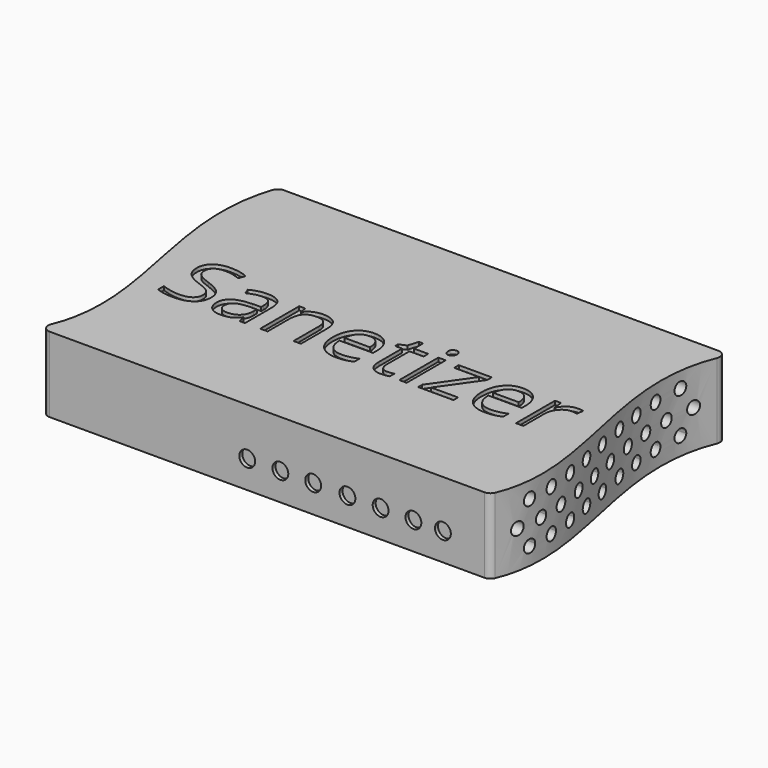
from build123d import *

# Parameters (mm, degrees)
F1_DEPTH      = 25.4
F2_R          = 2.54
F3_TEXT_SIZE  = 30.7263651242
F4_DEPTH      = 1.27
F5_R          = 2.1391280129
F6_DEPTH      = 87.376
F6_DEPTH_BACK = 113.538
F7_W          = 14.690361917
F7_H          = 8.7442630902
F7_W_2        = 13.8159319758
F7_W_3        = 14.3405906856
F7_W_4        = 15.2150169015
F7_W_5        = 12.766623171
F7_H_2        = 4.8967869952
F7_W_6        = 21.1611157283
F7_R          = 3.9572028388
F8_DEPTH      = 7.62
F9_R          = 2.6752298393
F10_DEPTH     = 1.27


# Not quite as in the source:
# - Text() gives the source's letters only with a copy of the font that has no kerning and outlines rounded to 1/6400 em; it was checked with that copy


with BuildPart() as f1:
    # F0 (on Top) → F1 (new body)
    with BuildSketch(Plane.XY):
        with BuildLine():
            add(Edge.make_bspline(
                [(-45.4201986909, 65.6159471944), (-58.06190148, 32.6160974801), (-29.9053769559, -7.6075084507), (-45.4201986909, -35.9840528056)],
                knots=[0, 0, 0, 0, 101.6, 101.6, 101.6, 101.6], degree=3))
            Line((-45.4201986909, -35.9840528056), (106.9798013091, -35.9840528056))
            add(Edge.make_bspline(
                [(106.9798013091, 65.6159471944), (90.3426812113, 34.0577052146), (120.670825243, -8.1321643665), (106.9798013091, -35.9840528056)],
                knots=[0, 0, 0, 0, 101.6, 101.6, 101.6, 101.6], degree=3))
            Line((106.9798013091, 65.6159471944), (-45.4201986909, 65.6159471944))
        make_face()
    extrude(amount=F1_DEPTH)

    # F2
    f2_edges = [f1.edges().sort_by_distance(p)[0] for p in [
        (106.979801, 65.615947, 12.7),
        (-45.420199, -35.984053, 12.7),
        (-45.420199, 65.615947, 12.7),
        (106.979801, -35.984053, 12.7),
    ]]
    fillet(f2_edges, radius=F2_R)

    # F3 (on face) → F4 (cut)
    with BuildSketch(Plane.XY.offset(25.4)):
        with Locations((-35.7243866998, 0)):
            Text('Sanetizer', F3_TEXT_SIZE, font='Open Sans', text_align=(TextAlign.LEFT, TextAlign.BOTTOM))
    extrude(amount=-F4_DEPTH, mode=Mode.SUBTRACT)

    # F5 (on Right) → F6 (cut, two sides)
    with BuildSketch(Plane.YZ) as f6_sk:
        with BuildLine():
            ThreePointArc((-25.4598658399, 12.6498732716), (-27.5989938527, 14.7890012844), (-29.7381218656, 12.6498732716))
            Line((-29.7381218656, 12.6498732716), (-25.4598658399, 12.6498732716))
        make_face()
        with BuildLine():
            ThreePointArc((57.1315141528, 12.8702148795), (54.882068538, 15.0064963877), (52.8646365703, 12.6498732716))
            Line((52.8646365703, 12.6498732716), (57.1201357096, 12.6498732716))
            ThreePointArc((57.1201357096, 12.6498732716), (57.1286676481, 12.7598972776), (57.1315141528, 12.8702148795))
        make_face()
        with BuildLine():
            Line((57.1201357096, 12.6498732716), (52.8646365703, 12.6498732716))
            ThreePointArc((52.8646365703, 12.6498732716), (54.9923861399, 10.7310868667), (57.1201357096, 12.6498732716))
        make_face()
        with BuildLine():
            ThreePointArc((47.2161371394, 12.6498732716), (45.0770091265, 14.7890012844), (42.9378811137, 12.6498732716))
            Line((42.9378811137, 12.6498732716), (47.2161371394, 12.6498732716))
        make_face()
        with BuildLine():
            Line((47.2161371394, 12.6498732716), (42.9378811137, 12.6498732716))
            ThreePointArc((42.9378811137, 12.6498732716), (45.0770091265, 10.5107452587), (47.2161371394, 12.6498732716))
        make_face()
        with BuildLine():
            ThreePointArc((38.182130283, 12.6498732716), (36.0430022702, 14.7890012844), (33.9038742573, 12.6498732716))
            Line((33.9038742573, 12.6498732716), (38.182130283, 12.6498732716))
        make_face()
        with BuildLine():
            Line((38.182130283, 12.6498732716), (33.9038742573, 12.6498732716))
            ThreePointArc((33.9038742573, 12.6498732716), (36.0430022702, 10.5107452587), (38.182130283, 12.6498732716))
        make_face()
        with BuildLine():
            ThreePointArc((29.2582979559, 12.6498732716), (27.119169943, 14.7890012844), (24.9800419302, 12.6498732716))
            Line((24.9800419302, 12.6498732716), (29.2582979559, 12.6498732716))
        make_face()
        with BuildLine():
            Line((29.2582979559, 12.6498732716), (24.9800419302, 12.6498732716))
            ThreePointArc((24.9800419302, 12.6498732716), (27.119169943, 10.5107452587), (29.2582979559, 12.6498732716))
        make_face()
        with BuildLine():
            ThreePointArc((19.6855726131, 12.6498732716), (17.5464468775, 14.7858799568), (15.4073211419, 12.6498732716))
            Line((15.4073211419, 12.6498732716), (19.6855726131, 12.6498732716))
        make_face()
        with BuildLine():
            Line((19.6855726131, 12.6498732716), (15.4073211419, 12.6498732716))
            ThreePointArc((15.4073211419, 12.6498732716), (17.5448862133, 10.5076245004), (19.6855748904, 12.646751944))
            ThreePointArc((19.6855748904, 12.646751944), (19.6855743211, 12.6483126082), (19.6855726131, 12.6498732716))
        make_face()
        with BuildLine():
            ThreePointArc((10.6515657568, 12.6498732716), (8.5124400211, 14.7858799568), (6.3733142855, 12.6498732716))
            Line((6.3733142855, 12.6498732716), (10.6515657568, 12.6498732716))
        make_face()
        with BuildLine():
            Line((10.6515657568, 12.6498732716), (6.3733142855, 12.6498732716))
            ThreePointArc((6.3733142855, 12.6498732716), (8.5108793569, 10.5076245004), (10.651568034, 12.646751944))
            ThreePointArc((10.651568034, 12.646751944), (10.6515674647, 12.6483126082), (10.6515657568, 12.6498732716))
        make_face()
        with BuildLine():
            ThreePointArc((1.7277334296, 12.6498732716), (-0.411392306, 14.7858799568), (-2.5505180416, 12.6498732716))
            Line((-2.5505180416, 12.6498732716), (1.7277334296, 12.6498732716))
        make_face()
        with BuildLine():
            Line((1.7277334296, 12.6498732716), (-2.5505180416, 12.6498732716))
            ThreePointArc((-2.5505180416, 12.6498732716), (-0.4129529702, 10.5076245004), (1.7277357069, 12.646751944))
            ThreePointArc((1.7277357069, 12.646751944), (1.7277351376, 12.6483126082), (1.7277334296, 12.6498732716))
        make_face()
        with BuildLine():
            ThreePointArc((-7.5020266564, 12.6498732716), (-9.6411546692, 14.7890012844), (-11.7802826821, 12.6498732716))
            Line((-11.7802826821, 12.6498732716), (-7.5020266564, 12.6498732716))
        make_face()
        with BuildLine():
            Line((-7.5020266564, 12.6498732716), (-11.7802826821, 12.6498732716))
            ThreePointArc((-11.7802826821, 12.6498732716), (-9.6411546692, 10.5107452587), (-7.5020266564, 12.6498732716))
        make_face()
        with BuildLine():
            ThreePointArc((-16.5360335127, 12.6498732716), (-18.6751615256, 14.7890012844), (-20.8142895385, 12.6498732716))
            Line((-20.8142895385, 12.6498732716), (-16.5360335127, 12.6498732716))
        make_face()
        with BuildLine():
            Line((-16.5360335127, 12.6498732716), (-20.8142895385, 12.6498732716))
            ThreePointArc((-20.8142895385, 12.6498732716), (-18.6751615256, 10.5107452587), (-16.5360335127, 12.6498732716))
        make_face()
        with BuildLine():
            Line((-25.4598658399, 12.6498732716), (-29.7381218656, 12.6498732716))
            ThreePointArc((-29.7381218656, 12.6498732716), (-27.5989938527, 10.5107452587), (-25.4598658399, 12.6498732716))
        make_face()
        with BuildLine():
            ThreePointArc((-21.1085888514, 5.9294542298), (-23.2473574579, 8.0293712339), (-25.3861260644, 5.9294542298))
            Line((-25.3861260644, 5.9294542298), (-21.1085888514, 5.9294542298))
        make_face()
        with BuildLine():
            ThreePointArc((52.5593182205, 6.110584829), (50.3295434849, 8.2477913766), (48.288744604, 5.9294542298))
            Line((48.288744604, 5.9294542298), (52.5516358113, 5.9294542298))
            ThreePointArc((52.5516358113, 5.9294542298), (52.5573967552, 6.0199381062), (52.5593182205, 6.110584829))
        make_face()
        with BuildLine():
            Line((52.5516358113, 5.9294542298), (48.288744604, 5.9294542298))
            ThreePointArc((48.288744604, 5.9294542298), (50.4201902077, 3.9714568161), (52.5516358113, 5.9294542298))
        make_face()
        with BuildLine():
            ThreePointArc((42.6435818008, 5.9294542298), (40.5048131943, 8.0293712339), (38.3660445878, 5.9294542298))
            Line((38.3660445878, 5.9294542298), (42.6435818008, 5.9294542298))
        make_face()
        with BuildLine():
            Line((42.6435818008, 5.9294542298), (38.3660445878, 5.9294542298))
            ThreePointArc((38.3660445878, 5.9294542298), (40.4852068664, 3.7512050617), (42.6439412071, 5.8902432211))
            ThreePointArc((42.6439412071, 5.8902432211), (42.6438513537, 5.909849549), (42.6435818008, 5.9294542298))
        make_face()
        with BuildLine():
            ThreePointArc((33.6095749444, 5.9294542298), (31.4708063379, 8.0293712339), (29.3320377314, 5.9294542298))
            Line((29.3320377314, 5.9294542298), (33.6095749444, 5.9294542298))
        make_face()
        with BuildLine():
            Line((33.6095749444, 5.9294542298), (29.3320377314, 5.9294542298))
            ThreePointArc((29.3320377314, 5.9294542298), (31.45120001, 3.7512050617), (33.6099343508, 5.8902432211))
            ThreePointArc((33.6099343508, 5.8902432211), (33.6098444973, 5.909849549), (33.6095749444, 5.9294542298))
        make_face()
        with BuildLine():
            ThreePointArc((24.6857426173, 5.9294542298), (22.5469740108, 8.0293712339), (20.4082054043, 5.9294542298))
            Line((20.4082054043, 5.9294542298), (24.6857426173, 5.9294542298))
        make_face()
        with BuildLine():
            Line((24.6857426173, 5.9294542298), (20.4082054043, 5.9294542298))
            ThreePointArc((20.4082054043, 5.9294542298), (22.5273676829, 3.7512050617), (24.6861020236, 5.8902432211))
            ThreePointArc((24.6861020236, 5.8902432211), (24.6860121701, 5.909849549), (24.6857426173, 5.9294542298))
        make_face()
        with BuildLine():
            ThreePointArc((15.1129600486, 5.9294542298), (12.9742509453, 8.0262499063), (10.8355418419, 5.9294542298))
            Line((10.8355418419, 5.9294542298), (15.1129600486, 5.9294542298))
        make_face()
        with BuildLine():
            Line((15.1129600486, 5.9294542298), (10.8355418419, 5.9294542298))
            ThreePointArc((10.8355418419, 5.9294542298), (12.9530837408, 3.7480986106), (15.1133789581, 5.8871218935))
            ThreePointArc((15.1133789581, 5.8871218935), (15.1132742282, 5.9082890979), (15.1129600486, 5.9294542298))
        make_face()
        with BuildLine():
            ThreePointArc((6.0789531922, 5.9294542298), (3.9402440889, 8.0262499063), (1.8015349855, 5.9294542298))
            Line((1.8015349855, 5.9294542298), (6.0789531922, 5.9294542298))
        make_face()
        with BuildLine():
            Line((6.0789531922, 5.9294542298), (1.8015349855, 5.9294542298))
            ThreePointArc((1.8015349855, 5.9294542298), (3.9190768844, 3.7480986106), (6.0793721017, 5.8871218935))
            ThreePointArc((6.0793721017, 5.8871218935), (6.0792673718, 5.9082890979), (6.0789531922, 5.9294542298))
        make_face()
        with BuildLine():
            ThreePointArc((-2.8448791349, 5.9294542298), (-4.9835882382, 8.0262499063), (-7.1222973416, 5.9294542298))
            Line((-7.1222973416, 5.9294542298), (-2.8448791349, 5.9294542298))
        make_face()
        with BuildLine():
            Line((-2.8448791349, 5.9294542298), (-7.1222973416, 5.9294542298))
            ThreePointArc((-7.1222973416, 5.9294542298), (-5.0047554427, 3.7480986106), (-2.8444602254, 5.8871218935))
            ThreePointArc((-2.8444602254, 5.8871218935), (-2.8445649553, 5.9082890979), (-2.8448791349, 5.9294542298))
        make_face()
        with BuildLine():
            ThreePointArc((-12.074581995, 5.9294542298), (-14.2133506015, 8.0293712339), (-16.352119208, 5.9294542298))
            Line((-16.352119208, 5.9294542298), (-12.074581995, 5.9294542298))
        make_face()
        with BuildLine():
            Line((-12.074581995, 5.9294542298), (-16.352119208, 5.9294542298))
            ThreePointArc((-16.352119208, 5.9294542298), (-14.2329569294, 3.7512050617), (-12.0742225886, 5.8902432211))
            ThreePointArc((-12.0742225886, 5.8902432211), (-12.0743124421, 5.909849549), (-12.074581995, 5.9294542298))
        make_face()
        with BuildLine():
            Line((-21.1085888514, 5.9294542298), (-25.3861260644, 5.9294542298))
            ThreePointArc((-25.3861260644, 5.9294542298), (-23.2669637858, 3.7512050617), (-21.108229445, 5.8902432211))
            ThreePointArc((-21.108229445, 5.8902432211), (-21.1083192985, 5.909849549), (-21.1085888514, 5.9294542298))
        make_face()
        with Locations((-14.2133506015, 19.9211463332)):
            Circle(F5_R)
        with Locations((-23.2473574579, 19.9211463332)):
            Circle(F5_R)
        with Locations((-4.9835882382, 19.9180250056)):
            Circle(F5_R)
        with Locations((12.9742509453, 19.9180250056)):
            Circle(F5_R)
        with Locations((3.9402440889, 19.9180250056)):
            Circle(F5_R)
        with Locations((22.5469740108, 19.9211463332)):
            Circle(F5_R)
        with Locations((40.5048131943, 19.9211463332)):
            Circle(F5_R)
        with Locations((31.4708063379, 19.9211463332)):
            Circle(F5_R)
        with Locations((50.4201902077, 20.1414879411)):
            Circle(F5_R)
    extrude(amount=-F6_DEPTH, mode=Mode.SUBTRACT)
    extrude(f6_sk.sketch, amount=F6_DEPTH_BACK, mode=Mode.SUBTRACT)

    # F7 (on face) → F8 (cut)
    with BuildSketch(Plane(origin=(0, 65.6159471944, 0), x_dir=(-1, 0, 0), z_dir=(0, 1, 0))):
        with Locations((-90.1482515037, 11.45498408)):
            Rectangle(F7_W, F7_H)
        with Locations((-75.8951045573, 11.45498408)):
            Rectangle(F7_W_2, F7_H)
        with Locations((-61.8168432266, 11.45498408)):
            Rectangle(F7_W_3, F7_H)
        with Locations((-47.4762525409, 11.45498408)):
            Rectangle(F7_W_3, F7_H)
        with Locations((-26.5774652362, 11.45498408)):
            Rectangle(F7_W_4, F7_H)
        with Locations((-4.8916939413, 9.5312460326)):
            Rectangle(F7_W_5, F7_H_2)
        with Locations((15.0452242233, 9.5312460326)):
            Rectangle(F7_W_6, F7_H_2)
        with Locations((35.594239831, 9.5312460326)):
            Circle(F7_R)
    extrude(amount=-F8_DEPTH, mode=Mode.SUBTRACT)

    # F9 (on face) → F10 (cut)
    with BuildSketch(Plane.XZ.offset(35.9840528056)):
        with Locations((36.4584811032, 9.3563608825)):
            Circle(F9_R)
        with Locations((25.2725430206, 9.3563608825)):
            Circle(F9_R)
        with Locations((47.5345365703, 9.3563608825)):
            Circle(F9_R)
        with Locations((70.2854409441, 9.3563608825)):
            Circle(F9_R)
        with Locations((59.0995028615, 9.3563608825)):
            Circle(F9_R)
        with Locations((81.3614964112, 9.3563608825)):
            Circle(F9_R)
        with Locations((91.3224592805, 9.3563608825)):
            Circle(F9_R)
    extrude(amount=-F10_DEPTH, mode=Mode.SUBTRACT)


solid = f1.part
